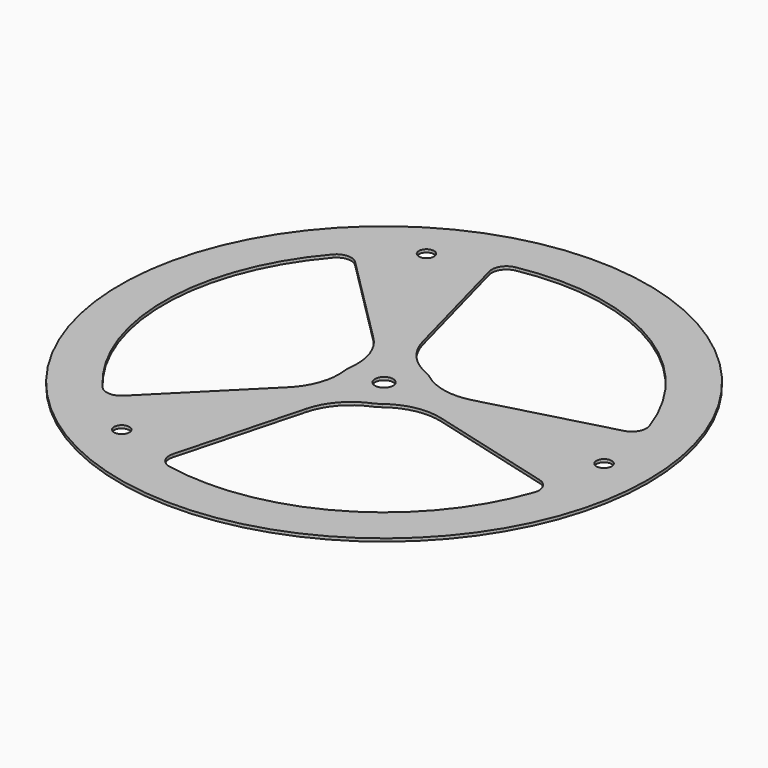
from build123d import *

# Parameters (mm, degrees)
F0_R            = 90
F0_R_2          = 3.1
F1_DEPTH        = 1
F3_DEPTH        = 12.5
F3_COPIES_COUNT = 3
F4_R            = 2.6
F5_DEPTH        = 25
F5_COPIES_COUNT = 3
F6_R            = 5
F7_R            = 20


# Not quite as in the source:
# - a pattern or mirror of a feature is missing from the dataset's text; its kind, count and spacing are read off the source's solid


with BuildPart() as f1:
    # F0 (on Top) → F1 (new body)
    with BuildSketch(Plane.XY):
        Circle(F0_R)
        Circle(F0_R_2, mode=Mode.SUBTRACT)
    extrude(amount=-F1_DEPTH)

    # F2 (on Top) → F3 (cut, symmetric)
    with BuildSketch(Plane.XY):
        with BuildLine():
            ThreePointArc((-3.2352380638, 12.0740728286), (6.25, 10.8253175473), (12.0740728286, 3.2352380638))
            Line((12.0740728286, 3.2352380638), (72.4444369717, 19.4114283827))
            ThreePointArc((72.4444369717, 19.4114283827), (37.5, 64.9519052838), (-19.4114283827, 72.4444369717))
            Line((-19.4114283827, 72.4444369717), (-3.2352380638, 12.0740728286))
        make_face()
    f3 = extrude(amount=F3_DEPTH, both=True, mode=Mode.SUBTRACT)

    # F3_copies: F3 ×3 about axis
    f3_copies_axis = Axis((0, 0, 0), (0, 0, 1))
    for i in range(1, F3_COPIES_COUNT):
        add(f3.rotate(f3_copies_axis, i * 360 / F3_COPIES_COUNT), mode=Mode.SUBTRACT)

    # F4 (on Top) → F5 (cut)
    with BuildSketch(Plane.XY):
        with Locations((75, 0)):
            Circle(F4_R)
    f5 = extrude(amount=-F5_DEPTH, mode=Mode.SUBTRACT)

    # F5_copies: F5 ×3 about axis
    f5_copies_axis = Axis((0, 0, 0), (0, 0, 1))
    for i in range(1, F5_COPIES_COUNT):
        add(f5.rotate(f5_copies_axis, i * 360 / F5_COPIES_COUNT), mode=Mode.SUBTRACT)

    # F6
    f6_edges = [f1.edges().sort_by_distance(p)[0] for p in [
        (-19.411428, 72.444437, -0.5),
        (72.444437, 19.411428, -0.5),
        (-53.033009, 53.033009, -0.5),
        (-53.033009, -53.033009, -0.5),
        (-19.411428, -72.444437, -0.5),
        (72.444437, -19.411428, -0.5),
    ]]
    fillet(f6_edges, radius=F6_R)

    # F7
    f7_edges = [f1.edges().sort_by_distance(p)[0] for p in [
        (12.074073, 3.235238, -0.5),
        (-3.235238, 12.074073, -0.5),
        (-8.838835, 8.838835, -0.5),
        (-8.838835, -8.838835, -0.5),
        (-3.235238, -12.074073, -0.5),
        (12.074073, -3.235238, -0.5),
    ]]
    fillet(f7_edges, radius=F7_R)


solid = f1.part
